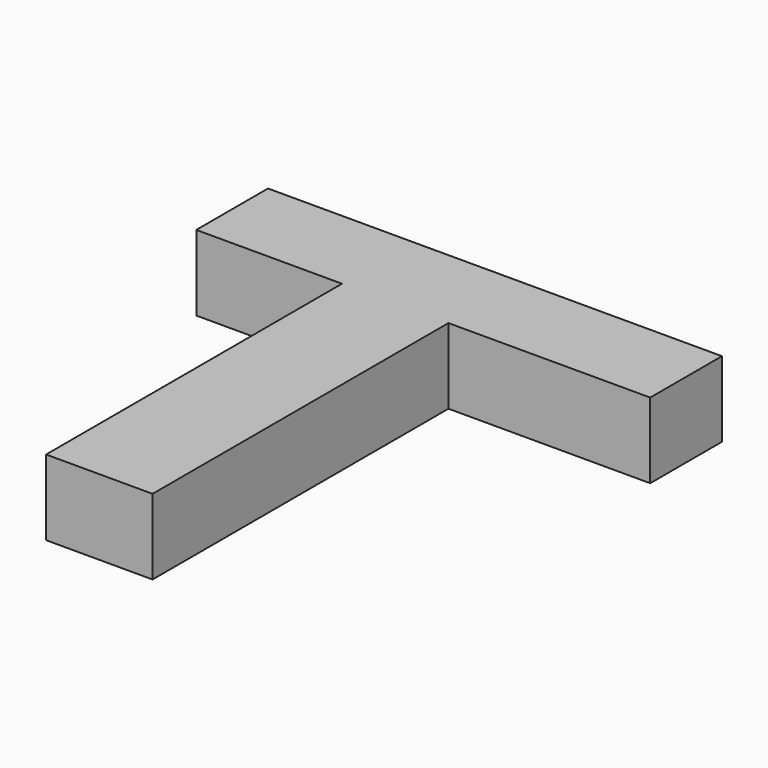
from build123d import *

# Parameters (mm, degrees)
F0_W     = 7.1707069874
F0_H     = 24.9087717384
F1_DEPTH = 5.08


# Not quite as in the source:
# - the program builds the solid bodies; features that only make, move or delete a surface that nothing else refers to are left out


with BuildPart() as f1:
    # F0 (on Top) → F1 (new body)
    with BuildSketch(Plane.XY):
        with Locations((-32.4568860233, 21.1347164586)):
            Rectangle(F0_W, F0_H)
        Polygon((-15.2849294245, 39.6275930107), (-45.8547882736, 39.6275930107), (-45.8547882736, 33.5891023278), (-36.042239517, 33.5891023278), (-28.8715325296, 33.5891023278), (-15.2849294245, 33.5891023278), align=None)
    extrude(amount=F1_DEPTH)


solid = f1.part
